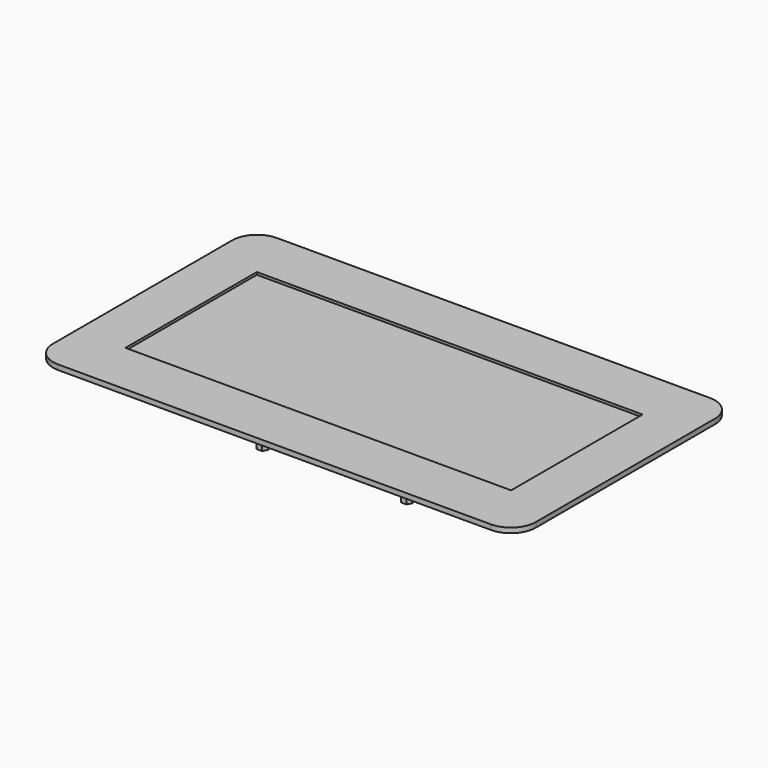
from build123d import *

# Parameters (mm, degrees)
F1_DEPTH = 2
F2_W     = 155
F2_H     = 66
F3_DEPTH = 1
F4_R     = 1.4
F5_DEPTH = 5.1
F6_W     = 65
F6_H     = 56
F6_R     = 1.4
F7_DEPTH = 1.6
F8_R     = 1.4
F9_DEPTH = 14.4


with BuildPart() as f1:
    # F0 (on Top) → F1 (new body)
    with BuildSketch(Plane.XY):
        with BuildLine():
            Line((87, 55), (-87, 55))
            ThreePointArc((-87, 55), (-94.0710678119, 52.0710678119), (-97, 45))
            Line((-97, 45), (-97, -45))
            ThreePointArc((-97, -45), (-94.0710678119, -52.0710678119), (-87, -55))
            Line((-87, -55), (87, -55))
            ThreePointArc((87, -55), (94.0710678119, -52.0710678119), (97, -45))
            Line((97, -45), (97, 45))
            ThreePointArc((97, 45), (94.0710678119, 52.0710678119), (87, 55))
        make_face()
    extrude(amount=F1_DEPTH)

    # F2 (on face) → F3 (cut)
    with BuildSketch(Plane.XY.offset(2)):
        Rectangle(F2_W, F2_H)
    extrude(amount=-F3_DEPTH, mode=Mode.SUBTRACT)

    # F4 (on face) → F5 (join)
    with BuildSketch(Plane(origin=(0, 0, 0), x_dir=(1, 0, 0), z_dir=(0, 0, -1))):
        with Locations((-29, 24.5)):
            Circle(F4_R)
        with Locations((-29, -24.5)):
            Circle(F4_R)
        with Locations((29, -24.5)):
            Circle(F4_R)
        with Locations((29, 24.5)):
            Circle(F4_R)
    extrude(amount=F5_DEPTH)


with BuildPart() as f7:
    # F6 (on face) → F7 (new body)
    with BuildSketch(Plane(origin=(0, 0, -5.1), x_dir=(1, 0, 0), z_dir=(0, 0, -1))):
        Rectangle(F6_W, F6_H)
        with Locations((-29, -24.5)):
            Circle(F6_R, mode=Mode.SUBTRACT)
        with Locations((29, -24.5)):
            Circle(F6_R, mode=Mode.SUBTRACT)
        with Locations((-29, 24.5)):
            Circle(F6_R, mode=Mode.SUBTRACT)
        with Locations((29, 24.5)):
            Circle(F6_R, mode=Mode.SUBTRACT)
    extrude(amount=F7_DEPTH)


with BuildPart() as f9:
    # F8 (on face) → F9 (new body)
    with BuildSketch(Plane(origin=(0, 0, -6.7), x_dir=(1, 0, 0), z_dir=(0, 0, -1))):
        Polygon((-27.925, 22.6380453819), (-26.85, 24.5), (-27.925, 26.3619546181), (-30.075, 26.3619546181), (-31.15, 24.5), (-30.075, 22.6380453819), align=None)
        with Locations((-29, 24.5)):
            Circle(F8_R, mode=Mode.SUBTRACT)
    extrude(amount=F9_DEPTH)


with BuildPart() as f9b:
    # F8 (on face) → F9, piece 2 (new body)
    with BuildSketch(Plane(origin=(0, 0, -6.7), x_dir=(1, 0, 0), z_dir=(0, 0, -1))):
        Polygon((27.925, 26.3619546181), (26.85, 24.5), (27.925, 22.6380453819), (30.075, 22.6380453819), (31.15, 24.5), (30.075, 26.3619546181), align=None)
        with Locations((29, 24.5)):
            Circle(F8_R, mode=Mode.SUBTRACT)
    extrude(amount=F9_DEPTH)


with BuildPart() as f9c:
    # F8 (on face) → F9, piece 3 (new body)
    with BuildSketch(Plane(origin=(0, 0, -6.7), x_dir=(1, 0, 0), z_dir=(0, 0, -1))):
        Polygon((27.925, -22.6380453819), (26.85, -24.5), (27.925, -26.3619546181), (30.075, -26.3619546181), (31.15, -24.5), (30.075, -22.6380453819), align=None)
        with Locations((29, -24.5)):
            Circle(F8_R, mode=Mode.SUBTRACT)
    extrude(amount=F9_DEPTH)


with BuildPart() as f9d:
    # F8 (on face) → F9, piece 4 (new body)
    with BuildSketch(Plane(origin=(0, 0, -6.7), x_dir=(1, 0, 0), z_dir=(0, 0, -1))):
        Polygon((-27.925, -26.3619546181), (-26.85, -24.5), (-27.925, -22.6380453819), (-30.075, -22.6380453819), (-31.15, -24.5), (-30.075, -26.3619546181), align=None)
        with Locations((-29, -24.5)):
            Circle(F8_R, mode=Mode.SUBTRACT)
    extrude(amount=F9_DEPTH)


solid = Compound([f1.part, f7.part, f9.part, f9b.part, f9c.part, f9d.part])
